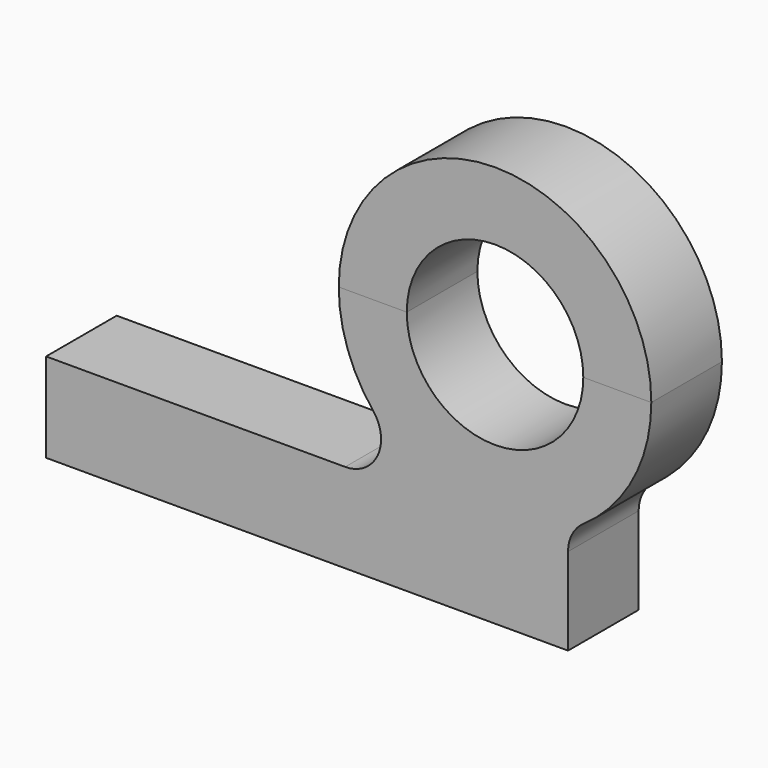
from build123d import *

# Parameters (mm, degrees)
F1_DEPTH = 25
F2_DEPTH = 25
F3_R     = 10.1752029192


# Not quite as in the source:
# - a feature names something its author has since deleted; it is built from what else it names


with BuildPart() as f1:
    # F0 (on Front) → F1 (new body)
    with BuildSketch(Plane.XZ):
        with BuildLine():
            Line((20.6833779812, -69.5540085435), (20.6833779812, -39.1374016096))
            ThreePointArc((20.6833779812, -39.1374016096), (10.6549466055, -42.9652236384), (0, -44.2666728981))
            Line((0, -44.2666728981), (-127.1657443379, -44.2666728981))
            Line((-127.1657443379, -44.2666728981), (-127.1657443379, -69.5540085435))
            Line((-127.1657443379, -69.5540085435), (20.6833779812, -69.5540085435))
        make_face()
    extrude(amount=F1_DEPTH)

    # F0 (on Front) → F2 (join)
    with BuildSketch(Plane.XZ):
        with BuildLine():
            Line((44.2666728981, 0), (25, 0))
            ThreePointArc((25, 0), (0, -25), (-25, 0))
            Line((-25, 0), (-44.2666728981, 0))
            ThreePointArc((-44.2666728981, 0), (-31.3012645868, -31.3012645868), (0, -44.2666728981))
            ThreePointArc((0, -44.2666728981), (10.6549466055, -42.9652236384), (20.6833779812, -39.1374016096))
            ThreePointArc((20.6833779812, -39.1374016096), (37.9151859879, -22.846815992), (44.2666728981, 0))
        make_face()
    extrude(amount=F2_DEPTH)

    # F3
    f3_edges = [f1.edges().sort_by_distance(p)[0] for p in [
        (0, -12.5, -44.266673),
        (20.683378, -12.5, -39.137402),
    ]]
    fillet(f3_edges, radius=F3_R)


with BuildPart() as f1b:
    # F0 (on Front) → F1, piece 2 (new body)
    with BuildSketch(Plane.XZ):
        with BuildLine():
            ThreePointArc((-25, 0), (0, 25), (25, 0))
            Line((25, 0), (44.2666728981, 0))
            ThreePointArc((44.2666728981, 0), (0, 44.2666728981), (-44.2666728981, 0))
            Line((-44.2666728981, 0), (-25, 0))
        make_face()
    extrude(amount=F1_DEPTH)


solid = Compound([f1.part, f1b.part])
